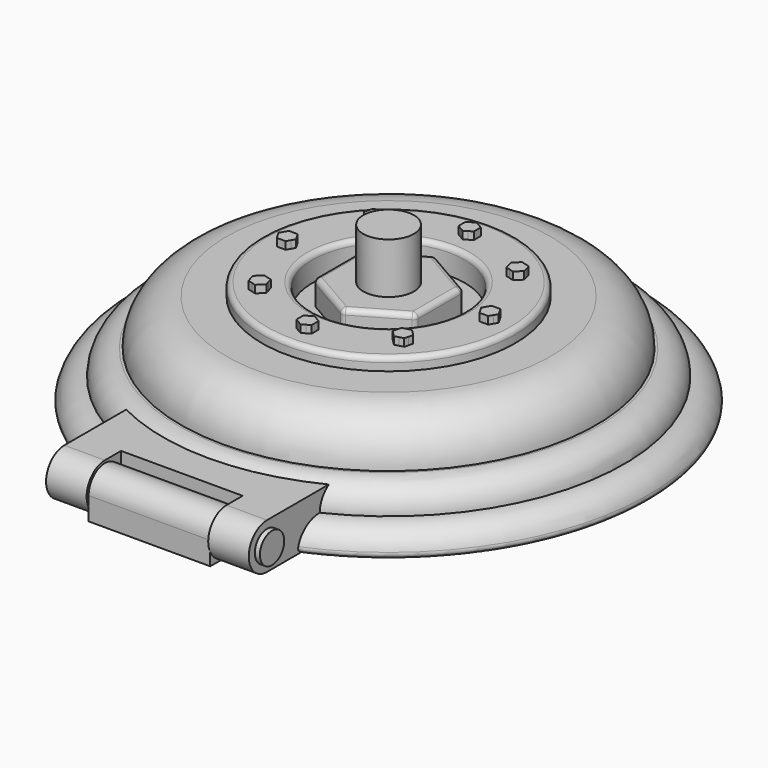
from build123d import *

# Parameters (mm, degrees)
F3_DEPTH  = 1
F4_R      = 0.2
F5_R      = 1
F6_DEPTH  = 2
F8_DEPTH  = 0.3
F9_COUNT  = 8
F11_DEPTH = 4
F12_W     = 4.8
F12_H     = 0.8
F12_H_2   = 4.2
F13_DEPTH = 1.8010001
F14_R     = 0.6
F15_DEPTH = 4.2
F17_DEPTH = 2.4


# Not quite as in the source:
# - a feature names something its author has since deleted; it is built from what else it names


with BuildPart() as f1:
    # F0 (on Right) → F1 (revolve)
    with BuildSketch(Plane.YZ):
        with BuildLine():
            Line((0, 3.3), (0, 0))
            Line((0, 0), (10.3, 0))
            ThreePointArc((10.3, 0), (10.0071067812, 0.7071067812), (9.3, 1))
            ThreePointArc((9.3, 1), (9.0071067812, 1.7071067812), (8.3, 2))
            Line((8.3, 2), (5, 2))
            Line((5, 2), (5, 4.3))
            Line((5, 4.3), (3, 4.3))
            Line((3, 4.3), (3, 3.3))
            Line((3, 3.3), (0, 3.3))
        make_face()
    revolve(axis=Axis((0, 0, 1.65), (0, 0, -1)))

    # F2 (on face) → F3 (join)
    with BuildSketch(Plane.XY.offset(3.3)):
        Polygon((2, 1.1547005384), (0, 2.3094010768), (-2, 1.1547005384), (-2, -1.1547005384), (0, -2.3094010768), (2, -1.1547005384), align=None)
    extrude(amount=F3_DEPTH)

    # F4
    f4_edges = [f1.edges().sort_by_distance(p)[0] for p in [
        (1, -1.732051, 4.3),
        (2, 0, 4.3),
        (1, 1.732051, 4.3),
        (-1, 1.732051, 4.3),
        (-2, 0, 4.3),
        (-1, -1.732051, 4.3),
        (0, -5, 4.3),
        (0, -3, 4.3),
        (0, -2.309401, 3.8),
        (-2, -1.154701, 3.8),
        (2, -1.154701, 3.8),
        (2, 1.154701, 3.8),
        (0, -10.3, 0),
        (0, 2.309401, 3.8),
        (-2, 1.154701, 3.8),
    ]]
    fillet(f4_edges, radius=F4_R)

    # F5 (on face) → F6 (join)
    with BuildSketch(Plane.XY.offset(4.3)):
        Circle(F5_R)
    extrude(amount=F6_DEPTH)



with BuildPart() as f8:
    # F7 (on face) → F8 (new body)
    with BuildSketch(Plane.XY.offset(4.3)):
        with BuildLine():
            Line((-0.3, 3.8267949192), (-0.1499999937, 3.7401923752))
            ThreePointArc((-0.1499999937, 3.7401923752), (-0.2598076193, 3.8499999969), (-0.3, 4))
            Line((-0.3, 4), (-0.3, 3.8267949192))
        make_face()
        with BuildLine():
            Line((0, 3.6535898385), (0.1500000107, 3.740192385))
            ThreePointArc((0.1500000107, 3.740192385), (9.8e-09, 3.7), (-0.1499999937, 3.7401923752))
            Line((-0.1499999937, 3.7401923752), (0, 3.6535898385))
        make_face()
        with BuildLine():
            Line((0.3, 3.8267949192), (0.3, 4))
            ThreePointArc((0.3, 4), (0.2598076242, 3.8500000053), (0.1500000107, 3.740192385))
            Line((0.1500000107, 3.740192385), (0.3, 3.8267949192))
        make_face()
        with BuildLine():
            ThreePointArc((-0.3, 4), (-0.2598076193, 4.1500000031), (-0.1499999937, 4.2598076248))
            Line((-0.1499999937, 4.2598076248), (-0.3, 4.1732050808))
            Line((-0.3, 4.1732050808), (-0.3, 4))
        make_face()
        with BuildLine():
            ThreePointArc((-0.1499999937, 4.2598076248), (1.96e-08, 4.3), (0.1500000276, 4.2598076052))
            Line((0.1500000276, 4.2598076052), (0, 4.3464101615))
            Line((0, 4.3464101615), (-0.1499999937, 4.2598076248))
        make_face()
        with BuildLine():
            ThreePointArc((0.1500000276, 4.2598076052), (0.2598076291, 4.1499999862), (0.3, 4))
            Line((0.3, 4), (0.3, 4.1732050808))
            Line((0.3, 4.1732050808), (0.1500000276, 4.2598076052))
        make_face()
        with BuildLine():
            ThreePointArc((0.1500000107, 3.740192385), (0.2598076242, 3.8500000053), (0.3, 4))
            ThreePointArc((0.3, 4), (0.2598076291, 4.1499999862), (0.1500000276, 4.2598076052))
            ThreePointArc((0.1500000276, 4.2598076052), (1.96e-08, 4.3), (-0.1499999937, 4.2598076248))
            ThreePointArc((-0.1499999937, 4.2598076248), (-0.2598076193, 4.1500000031), (-0.3, 4))
            ThreePointArc((-0.3, 4), (-0.2598076193, 3.8499999969), (-0.1499999937, 3.7401923752))
            ThreePointArc((-0.1499999937, 3.7401923752), (9.8e-09, 3.7), (0.1500000107, 3.740192385))
        make_face()
    extrude(amount=F8_DEPTH)


with BuildPart() as f1_1:
    add(f1.part)

    add(f8.part)  # F9 merges F8
    # F9: F8 ×8 about axis
    f9_axis = Axis((0, 0, 4.3), (0, 0, -1))
    for i in range(1, F9_COUNT):
        add(f8.part.rotate(f9_axis, i * 360 / F9_COUNT))

    # F10 (on Right) → F11 (join, symmetric)
    with BuildSketch(Plane.YZ):
        with BuildLine():
            Line((-11, 0), (-4, 0))
            Line((-4, 0), (-4, 1.8))
            Line((-4, 1.8), (-11, 1.8))
            ThreePointArc((-11, 1.8), (-11.9, 0.9), (-11, 0))
        make_face()
    extrude(amount=F11_DEPTH, both=True)

    # F12 (on face) → F13 (cut, through all)
    with BuildSketch(Plane.XY.offset(1.8)):
        with Locations((0, -10.6)):
            Rectangle(F12_W, F12_H)
        with Locations((0, -13.1)):
            Rectangle(F12_W, F12_H_2)
    extrude(amount=-F13_DEPTH, mode=Mode.SUBTRACT)

    # F14 (on Right) → F15 (join, symmetric)
    with BuildSketch(Plane.YZ):
        with Locations((-11, 0.9)):
            Circle(F14_R)
    extrude(amount=F15_DEPTH, both=True)

    # F16 (on Right) → F17 (join, symmetric)
    with BuildSketch(Plane.YZ):
        with BuildLine():
            Line((-10.2, 0), (-10.2, 0.9))
            ThreePointArc((-10.2, 0.9), (-11, 1.7), (-11.8, 0.9))
            Line((-11.8, 0.9), (-11.8, 0))
            Line((-11.8, 0), (-10.2, 0))
        make_face()
    extrude(amount=F17_DEPTH, both=True)

    # F18 (on Right) → F19 (revolve)
    with BuildSketch(Plane.YZ):
        with BuildLine():
            Line((4, 2), (8.2, 2))
            ThreePointArc((8.2, 2), (7.6727922061, 3.2727922061), (6.4, 3.8))
            Line((6.4, 3.8), (4, 3.8))
            Line((4, 3.8), (4, 2))
        make_face()
    revolve(axis=Axis((0, 0, 3), (0, 0, 1)))


solid = f1_1.part
